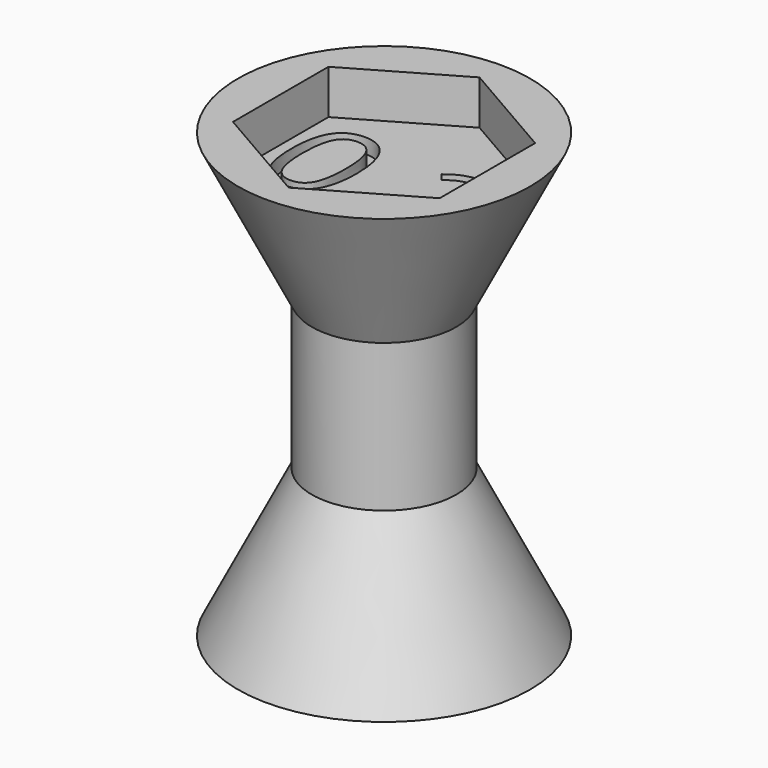
from build123d import *

# Parameters (mm, degrees)
F3_DEPTH     = 3
F4_TEXT_SIZE = 9.5018145826
F5_DEPTH     = 1


# Not quite as in the source:
# - Text() gives the source's letters only with a copy of the font that has no kerning and outlines rounded to 1/6400 em; it was checked with that copy


with BuildPart() as f1:
    # F0 (on Front) → F1 (revolve)
    with BuildSketch(Plane.XZ):
        Polygon((9.9, 15), (0, 15), (0, -15), (9.9, -15), (4.9, -5), (4.9, 5), align=None)
    revolve(axis=Axis((0, 0, 0), (0, 0, -1)))

    # F2 (on face) → F3 (cut)
    with BuildSketch(Plane.XY.offset(15)):
        Polygon((7, 4.0414518843), (0, 8.0829037687), (-7, 4.0414518843), (-7, -4.0414518843), (0, -8.0829037687), (7, -4.0414518843), align=None)
    extrude(amount=-F3_DEPTH, mode=Mode.SUBTRACT)

    # F4 (on face) → F5 (cut)
    with BuildSketch(Plane.XY.offset(12)):
        with Locations((-6.75, -3.4330531734)):
            Text('0.2', F4_TEXT_SIZE, font='Open Sans', text_align=(TextAlign.LEFT, TextAlign.BOTTOM))
    extrude(amount=-F5_DEPTH, mode=Mode.SUBTRACT)


solid = f1.part
